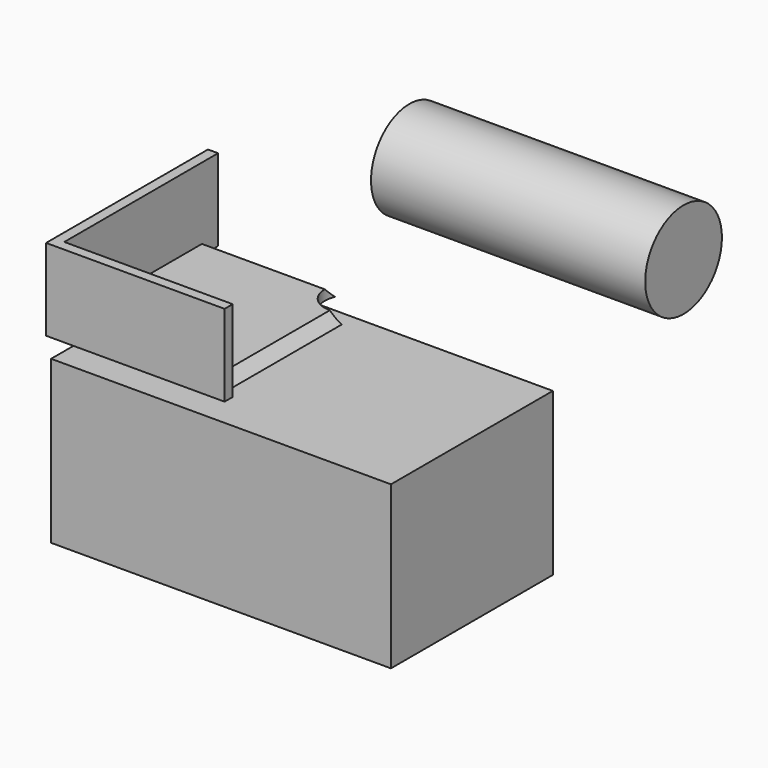
from build123d import *

# Parameters (mm, degrees)
F0_W          = 85.3199996054
F0_H          = 40.6800028868
F1_DEPTH      = 50.8
F0_W_2        = 44.8200013489
F0_H_2        = 20.5199993216
F2_T          = -2.54
F3_T1_DEPTH   = 55.3441509277
F3_T3_DEPTH   = 61.3241495789
F5_D          = 12.7
F6_R          = 12.039951047
F7_DEPTH      = 43.434
F7_DEPTH_BACK = 25.4


# Not quite as in the source:
# - a fillet or chamfer that OpenCascade refuses, or shapes differently, is made with other operations: its cross-section is extruded or revolved along the edge and cut away or added


with BuildPart() as f1:
    # F0 (on Front) → F1 (new body)
    with BuildSketch(Plane.XZ):
        with Locations((-10.0800003856, -27.810001513)):
            Rectangle(F0_W, F0_H)
    extrude(amount=F1_DEPTH)


with BuildPart() as f1b:
    # F0 (on Front) → F1, piece 2 (new body)
    with BuildSketch(Plane.XZ):
        with Locations((-31.5900007263, 7.4699998368)):
            Rectangle(F0_W_2, F0_H_2)
    extrude(amount=F1_DEPTH)

    # F2
    f2_openings = [f1b.faces().sort_by_distance(p)[0] for p in [
        (-31.590001, -25.4, 17.729999),
        (-31.590001, 0, 7.47),
        (-9.18, -25.4, 7.47),
    ]]
    offset(amount=F2_T, openings=f2_openings)

    # F3: chamfer of 5.08 on 2 edges, made by hand

    # F3_s2 → F3_t1 (cut)
    with BuildSketch(Plane.YZ.offset(-51.4600014007)):
        Polygon((0, -5.329999824), (-5.08, -0.249999824), (0, -0.249999824), align=None)
    extrude(amount=F3_T1_DEPTH, mode=Mode.SUBTRACT)

    # F3_s4 → F3_t3 (cut)
    with BuildSketch(Plane.XZ.offset(-13.0641495789)):
        Polygon((-9.1800000519, -5.329999824), (-14.2600000519, -0.249999824), (-9.1800000519, -0.249999824), align=None)
    extrude(amount=F3_T3_DEPTH, mode=Mode.SUBTRACT)

    # F5 (through all)
    with Locations(Plane.XY.offset(-0.249999824)):
        with Locations((-14.2600000519, -5.08)):
            Hole(F5_D / 2)


with BuildPart() as f7:
    # F6 (on Right) → F7 (new body, two sides)
    with BuildSketch(Plane.YZ) as f7_sk:
        with Locations((27.455566451, 13.9045361429)):
            Circle(F6_R)
    extrude(amount=F7_DEPTH)
    extrude(f7_sk.sketch, amount=-F7_DEPTH_BACK)


solid = Compound([f1.part, f1b.part, f7.part])
